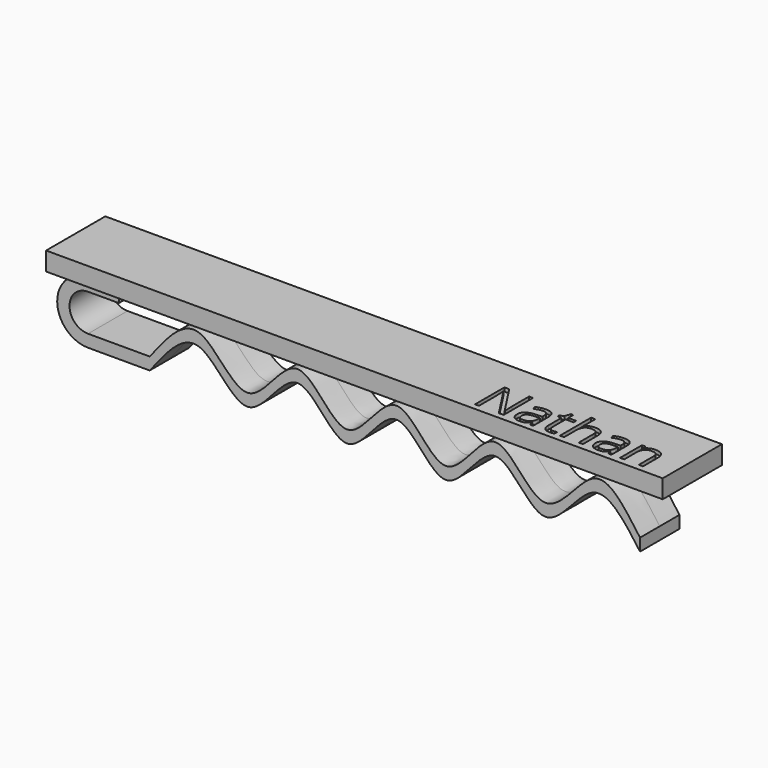
from build123d import *

# Parameters (mm, degrees)
F0_W         = 50
F0_H         = 6
F1_DEPTH     = 1.5
F3_DEPTH     = 2
F4_TEXT_SIZE = 4.1666666667
F5_DEPTH     = 0.3


# Not quite as in the source:
# - Text() gives the source's letters only with a copy of the font that has no kerning and outlines rounded to 1/6400 em; it was checked with that copy


with BuildPart() as f1:
    # F0 (on Top) → F1 (new body)
    with BuildSketch(Plane.XY):
        with Locations((0.728603825, 0)):
            Rectangle(F0_W, F0_H)
    extrude(amount=F1_DEPTH)

    # F2 (on Front) → F3 (join, symmetric)
    with BuildSketch(Plane.XZ):
        with BuildLine():
            Line((-21.6702353209, -1), (-21.6702353209, 0))
            ThreePointArc((-21.6702353209, 0), (-24.1702353209, -2.5), (-21.6702353209, -5))
            Line((-21.6702353209, -5), (-21.6702353209, -4))
            ThreePointArc((-21.6702353209, -4), (-23.1702353209, -2.5), (-21.6702353209, -1))
        make_face()
        with BuildLine():
            Line((-19.1702353209, 0), (-21.6702353209, 0))
            ThreePointArc((-21.6702353209, 0), (-20.5522013322, -0.2639320225), (-19.6702353209, -1))
            Line((-19.6702353209, -1), (-19.1702353209, -1))
            Line((-19.1702353209, -1), (-19.1702353209, 0))
        make_face()
        with BuildLine():
            ThreePointArc((-19.6702353209, -1), (-20.5522013322, -0.2639320225), (-21.6702353209, 0))
            Line((-21.6702353209, 0), (-21.6702353209, -1))
            Line((-21.6702353209, -1), (-19.6702353209, -1))
        make_face()
        with BuildLine():
            Line((-21.6702353209, -4), (-21.6702353209, -5))
            ThreePointArc((-21.6702353209, -5), (-20.5522013322, -4.7360679775), (-19.6702353209, -4))
            Line((-19.6702353209, -4), (-21.6702353209, -4))
        make_face()
        with BuildLine():
            ThreePointArc((-19.6702353209, -4), (-20.5522013322, -4.7360679775), (-21.6702353209, -5))
            Line((-21.6702353209, -5), (-16.6702353209, -5))
            Line((-16.6702353209, -5), (-16.6702353209, -4))
            Line((-16.6702353209, -4), (-19.6702353209, -4))
        make_face()
        with BuildLine():
            Line((-16.6702353209, -4), (-16.6702353209, -5))
            add(Edge.make_bspline(
                [(-16.6702353209, -5), (-15.3369020508, -3.2679551423), (-12.6702339992, 0.1961333993), (-8.6702398523, -7.7845341842), (-4.6702185171, 0.9420033374), (-0.6702980047, -7.9834791652), (3.3299986102, 0.9919133236), (7.3288916382, -7.9841741293), (11.3330229114, 0.9447831936), (15.3176047906, -7.7949586451), (19.3490540693, 0.1834145803), (21.8499493196, -3.2834501501), (23.0882172734, -5)],
                knots=[0, 0, 0, 0, 0.1001932872, 0.2003865745, 0.3005798617, 0.4007731489, 0.5009664362, 0.6011597234, 0.7013530106, 0.8015462979, 0.9017395851, 1, 1, 1, 1], degree=3))
            Line((23.0882172734, -5), (23.0882172734, -4))
            add(Edge.make_bspline(
                [(-16.6702353209, -4), (-15.3369089068, -2.2745677307), (-12.6702281185, 1.1991984576), (-8.6702501506, -6.7853430056), (-4.6701832046, 1.9421735646), (-0.6704289564, -6.9833512529), (3.3304871047, 1.9912314472), (7.3270686121, -6.9815745357), (11.3398265214, 1.9350666958), (15.2922133766, -6.7586922473), (19.4430434711, 1.0491690568), (21.6514973167, -2), (23.0882172734, -4)],
                knots=[0, 0, 0, 0, 0.1001932872, 0.2003865745, 0.3005798617, 0.4007731489, 0.5009664362, 0.6011597234, 0.7013530106, 0.8015462979, 0.9017395851, 1, 1, 1, 1], degree=3))
        make_face()
    extrude(amount=F3_DEPTH, both=True)

    # F4 (on face) → F5 (cut)
    with BuildSketch(Plane.XY.offset(1.5)):
        with Locations((9.7032132, -2.5)):
            Text('Nathan', F4_TEXT_SIZE, font='Open Sans', text_align=(TextAlign.LEFT, TextAlign.BOTTOM))
    extrude(amount=-F5_DEPTH, mode=Mode.SUBTRACT)


solid = f1.part
